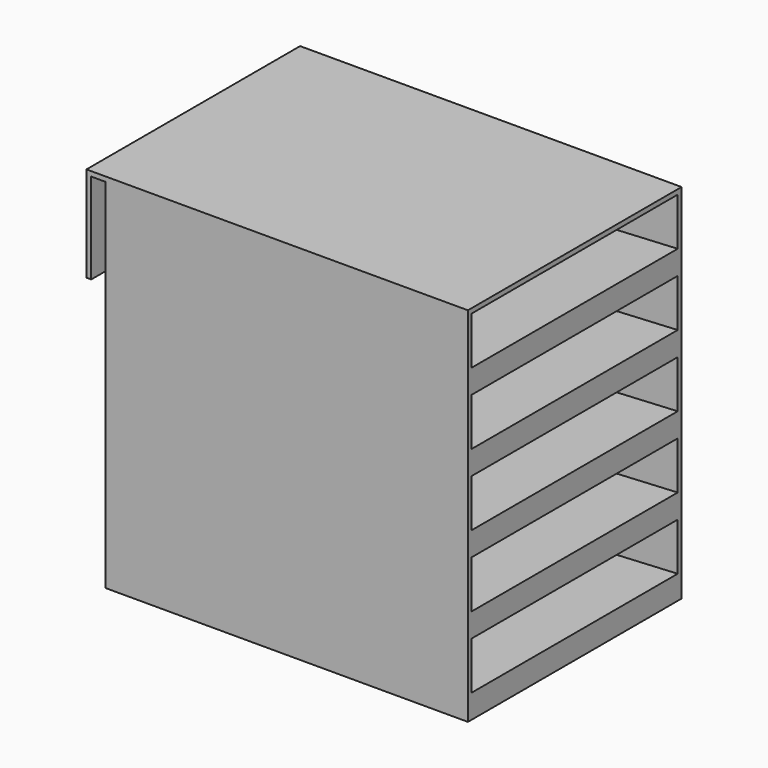
from build123d import *

# Parameters (mm, degrees)
F0_W           = 76
F0_H           = 76
F1_DEPTH       = 28
F2_W           = 54
F2_H           = 10
F5_W           = 56
F5_H           = 76
F6_DEPTH       = 1
F8_DEPTH       = 56
F9_TEXT_SIZE   = 8.9253324808
F9_TEXT_SIZE_2 = 9.2617753479
F9_TEXT_SIZE_3 = 9.3902593815
F9_TEXT_SIZE_4 = 9.6482923254
F9_TEXT_SIZE_5 = 10.8240379228
F10_DEPTH      = 1


# Not quite as in the source:
# - Text() gives the source's letters only with a copy of the font that has no kerning and outlines rounded to 1/6400 em; it was checked with that copy


with BuildPart() as f1:
    # F0 (on Front) → F1 (new body, symmetric)
    with BuildSketch(Plane.XZ):
        Rectangle(F0_W, F0_H)
    extrude(amount=F1_DEPTH, both=True)

    # F4: sweep along a path in F3
    with BuildLine(Plane.XZ.offset(28)) as f4_path:
        Line((38, 37), (-38, 33.0170087745))
    # F2 (on face) → F4 (sweep, cut)
    with BuildSketch(Plane.YZ.offset(38)):
        with Locations((0, 32)):
            Rectangle(F2_W, F2_H)
        with Locations((0, 17)):
            Rectangle(F2_W, F2_H)
        with Locations((0, 2)):
            Rectangle(F2_W, F2_H)
        with Locations((0, -13)):
            Rectangle(F2_W, F2_H)
        with Locations((0, -28)):
            Rectangle(F2_W, F2_H)
    sweep(path=f4_path.line, mode=Mode.SUBTRACT)

    # F5 (on face) → F6 (join)
    with BuildSketch(Plane(origin=(-38, 0, 0), x_dir=(0, -1, 0), z_dir=(-1, 0, 0))):
        Rectangle(F5_W, F5_H)
    extrude(amount=-F6_DEPTH)

    # F7 (on face) → F8 (join)
    with BuildSketch(Plane.XZ.offset(28)):
        Polygon((-38, 37), (-38, 38), (-42, 38), (-42, 18), (-41, 18), (-41, 37), align=None)
    extrude(amount=-F8_DEPTH)

    # F9 (on face) → F10 (join)
    with BuildSketch(Plane(origin=(0, 28, 0), x_dir=(-1, 0, 0), z_dir=(0, 1, 0))):
        with Locations((-30.6668113917, 28.5186786205)):
            Text('U', F9_TEXT_SIZE, font='Open Sans', text_align=(TextAlign.LEFT, TextAlign.BOTTOM))
        with Locations((-30.4371416569, 12.921391055)):
            Text('V', F9_TEXT_SIZE_2, font='Open Sans', text_align=(TextAlign.LEFT, TextAlign.BOTTOM))
        with Locations((-29.9739278853, -1.6359465662)):
            Text('W', F9_TEXT_SIZE_3, font='Open Sans', text_align=(TextAlign.LEFT, TextAlign.BOTTOM))
        with Locations((-29.9739278853, -16.6555196047)):
            Text('X/Y', F9_TEXT_SIZE_4, font='Open Sans', text_align=(TextAlign.LEFT, TextAlign.BOTTOM))
        with Locations((-29.9739278853, -33.0321379006)):
            Text('Z', F9_TEXT_SIZE_5, font='Open Sans', text_align=(TextAlign.LEFT, TextAlign.BOTTOM))
    extrude(amount=F10_DEPTH)


solid = f1.part
